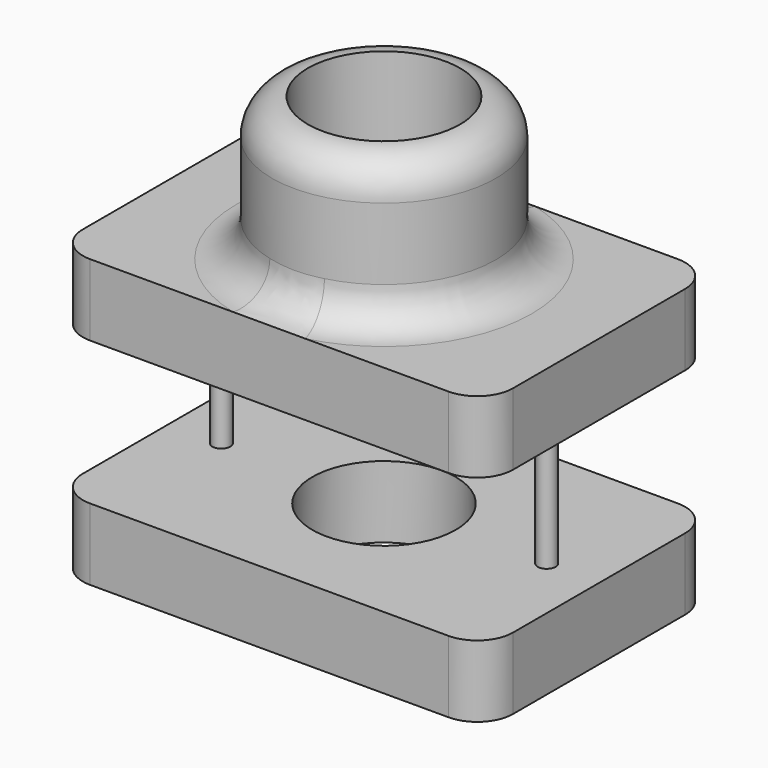
from build123d import *

# Parameters (mm, degrees)
F0_W     = 76.2
F0_H     = 50.8
F0_R     = 12.7
F1_DEPTH = 12.7
F2_R     = 6.35
F3_R     = 1.5875
F4_DEPTH = 25.4
F5_R     = 12.7
F6_DEPTH = 12.7
F7_W     = 6.35
F7_H     = 25.4
F9_R     = 6.34999


# Not quite as in the source:
# - a fillet or chamfer is up to 0.001 mm smaller than in the source, because OpenCascade refuses the exact size


with BuildPart() as f1:
    # F0 (on Top) → F1 (new body)
    with BuildSketch(Plane.XY):
        Rectangle(F0_W, F0_H)
        Circle(F0_R, mode=Mode.SUBTRACT)
    extrude(amount=F1_DEPTH)

    # F2
    f2_edges = [f1.edges().sort_by_distance(p)[0] for p in [
        (38.1, -25.4, 6.35),
        (38.1, 25.4, 6.35),
        (-38.1, -25.4, 6.35),
        (-38.1, 25.4, 6.35),
    ]]
    fillet(f2_edges, radius=F2_R)

    # F3 (on face) → F4 (join)
    with BuildSketch(Plane.XY.offset(12.7)):
        with Locations((-28.8149718722, 0)):
            Circle(F3_R)
        with Locations((28.8149718722, 0)):
            Circle(F3_R)
    extrude(amount=F4_DEPTH)

    # F5 (on face) → F6 (join)
    with BuildSketch(Plane.XY.offset(38.1)):
        with BuildLine():
            Line((-38.1, 19.05), (-38.1, -19.05))
            ThreePointArc((-38.1, -19.05), (-36.2401280605, -23.5401280605), (-31.75, -25.4))
            Line((-31.75, -25.4), (31.75, -25.4))
            ThreePointArc((31.75, -25.4), (36.2401280605, -23.5401280605), (38.1, -19.05))
            Line((38.1, -19.05), (38.1, 19.05))
            ThreePointArc((38.1, 19.05), (36.2401280605, 23.5401280605), (31.75, 25.4))
            Line((31.75, 25.4), (-31.75, 25.4))
            ThreePointArc((-31.75, 25.4), (-36.2401280605, 23.5401280605), (-38.1, 19.05))
        make_face()
        Circle(F5_R, mode=Mode.SUBTRACT)
    extrude(amount=F6_DEPTH)

    # F7 (on Front) → F8 (revolve)
    with BuildSketch(Plane.XZ):
        with Locations((-16.6624, 63.5)):
            Rectangle(F7_W, F7_H)
    revolve(axis=Axis((0, 0, 40.5965745449), (0, 0, 1)))

    # F9 (radius 6.35 in the source; OpenCascade refuses exactly that, so slightly less here)
    f9_edges = [f1.edges().sort_by_distance(p)[0] for p in [
        (19.8374, 0, 76.2),
        (19.8374, 0, 50.8),
    ]]
    fillet(f9_edges, radius=F9_R)


solid = f1.part
